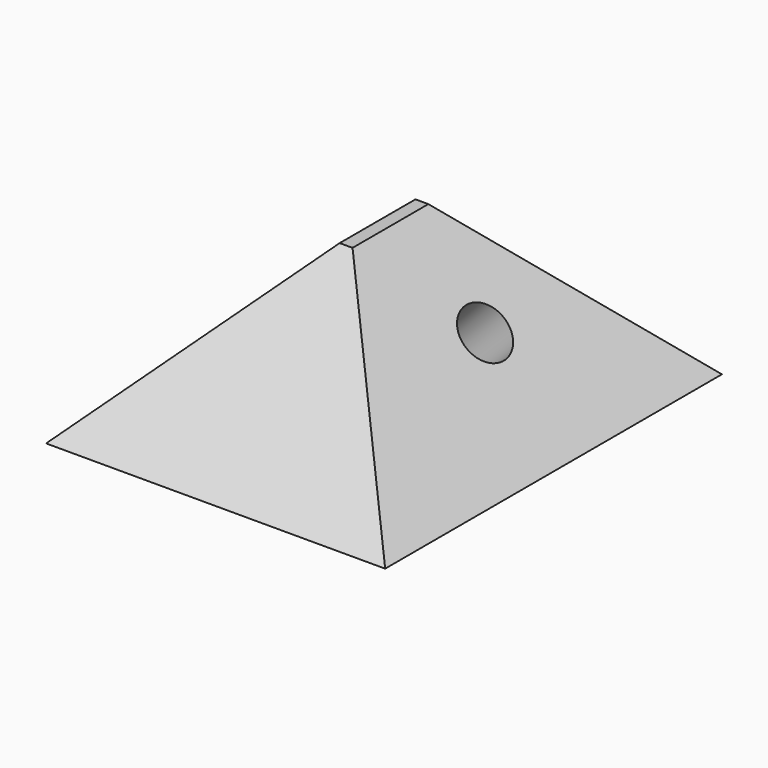
from build123d import *

# Parameters (mm, degrees)
F0_W     = 51.9770644605
F0_H     = 64.5220279694
F1_DEPTH = 25
F1_TAPER = 45
F2_R     = 4.0319564515
F3_DEPTH = 25


with BuildPart() as f1:
    # F0 (on Top) → F1 (new body)
    with BuildSketch(Plane.XY):
        with Locations((25.9885322303, 32.2610139847)):
            Rectangle(F0_W, F0_H)
    extrude(amount=F1_DEPTH, taper=F1_TAPER)

    # F2 (on face) → F3 (cut)
    with BuildSketch(Plane(origin=(25.9885322303, 0, 25.9885322303), x_dir=(0, 1, 0), z_dir=(0.7071067812, 0, 0.7071067812))):
        with Locations((35.5320125818, -18.2061810046)):
            Circle(F2_R)
    extrude(amount=-F3_DEPTH, mode=Mode.SUBTRACT)


solid = f1.part
